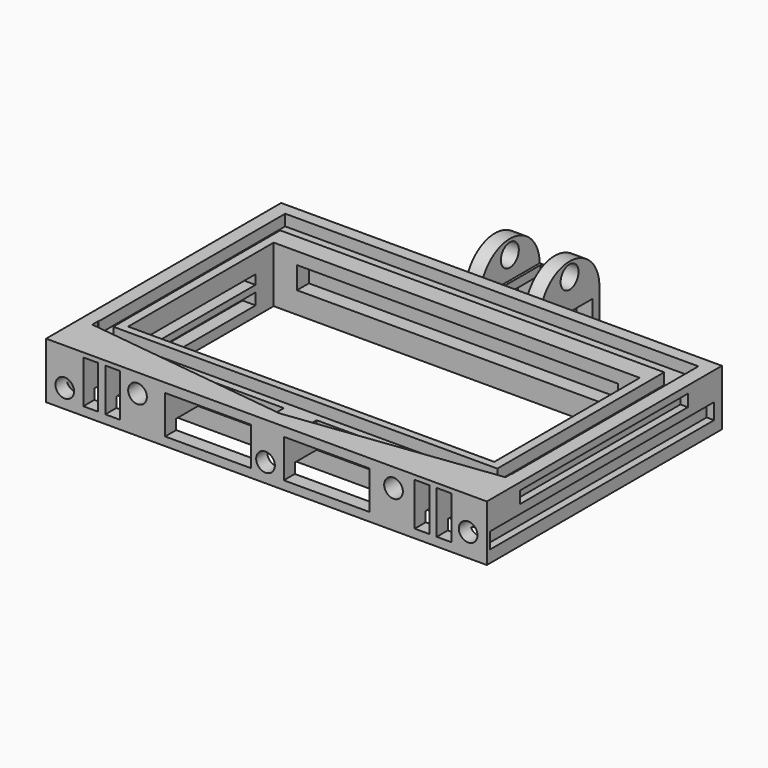
from build123d import *

# Parameters (mm, degrees)
F0_W      = 124.6
F0_H      = 61.9
F1_DEPTH  = 19.05
F2_W      = 4.953
F2_H      = 14.6315630991
F2_W_2    = 29.2449435338
F2_H_2    = 13.041177066
F2_W_3    = 29.159436468
F2_R      = 3.175
F3_DEPTH  = 13.97
F5_DEPTH  = 6.35
F6_W      = 12.7
F6_H      = 25.4
F7_DEPTH  = 12.7
F8_W      = 4.953
F8_H      = 71.0073517896
F9_DEPTH  = 3.81
F10_R     = 3.81
F11_DEPTH = 5.08
F13_DEPTH = 5.08
F14_DEPTH = 31.75
F16_W     = 13.5046280921
F16_H     = 23.5811583698
F17_DEPTH = 25.4
F18_W     = 19.2745104432
F18_H     = 5.7546193711
F19_DEPTH = 31.75
F20_W     = 14.9206416681
F20_H     = 4.7117811628
F21_DEPTH = 19.05
F22_W     = 51.0552711785
F22_H     = 10.1753515191
F22_W_2   = 51.412301138
F23_DEPTH = 12.7
F24_W     = 93.4092327952
F24_H     = 5.8380772825
F24_W_2   = 76.4692127705
F24_H_2   = 3.4473836422
F25_DEPTH = 2.54
F26_W     = 95.3170992434
F26_H     = 5.4240481682
F26_W_2   = 71.3913366199
F26_H_2   = 4.0845796466
F27_DEPTH = 2.54
F28_W     = 109.2679016292
F28_H     = 7.5388159603
F29_DEPTH = 5.08
F30_W     = 48.6481711268
F30_H     = 3.1835205168
F30_W_2   = 48.6969016492
F30_H_2   = 3.9205837529
F31_DEPTH = 5.08
F32_W     = 55.2894864231
F32_H     = 4.0775961243
F32_W_2   = 55.2933309227
F32_H_2   = 3.075633198
F33_DEPTH = 5.08


# Not quite as in the source:
# - a feature names something its author has since deleted; it is built from what else it names


with BuildPart() as f1:
    # F0 (on Top) → F1 (new body)
    with BuildSketch(Plane.XY):
        Polygon((-75.2904937168, 49.9057597088), (-75.2904937168, -50.0942402912), (-42.6597435957, -50.0942402912), (67.6151300783, -50.0942402912), (74.7095062832, -50.0942402912), (74.7095062832, 49.9057597088), (-0.2904937168, 49.9057597088), (-25.810170721, 49.9057597088), (-50.4447113996, 49.9057597088), align=None)
        with Locations((-0.2904937168, -0.0942402912)):
            Rectangle(F0_W, F0_H, mode=Mode.SUBTRACT)
    extrude(amount=F1_DEPTH)

    # F2 (on face) → F3 (cut)
    with BuildSketch(Plane.XZ.offset(50.0942402912)):
        with Locations((-60.1431414232, 10.2322226157)):
            Rectangle(F2_W, F2_H)
        with Locations((-52.6501414232, 10.2322226157)):
            Rectangle(F2_W, F2_H)
        with Locations((-20.147212787, 9.4370295992)):
            Rectangle(F2_W_2, F2_H_2)
        with Locations((20.1876896899, 9.4370295992)):
            Rectangle(F2_W_3, F2_H_2)
        with Locations((52.6363079239, 10.2322226157)):
            Rectangle(F2_W, F2_H)
        with Locations((60.1293079239, 10.2322226157)):
            Rectangle(F2_W, F2_H)
        with Locations((-44.1754937168, 12.7)):
            Circle(F2_R)
        with Locations((-0.6144937168, 6.35)):
            Circle(F2_R)
        with Locations((42.9465062832, 12.7)):
            Circle(F2_R)
        with Locations((68.3465062832, 7.8599134153)):
            Circle(F2_R)
        with Locations((-68.9404937168, 6.35)):
            Circle(F2_R)
    extrude(amount=-F3_DEPTH, mode=Mode.SUBTRACT)

    # F4 (on face) → F5 (cut)
    with BuildSketch(Plane(origin=(0, 0, 0), x_dir=(1, 0, 0), z_dir=(0, 0, -1))):
        Polygon((66.3145062832, 45.4020188174), (-67.0354937168, 45.4020188174), (-67.0354937168, 35.2429834301), (-61.1156715149, 35.2429834301), (60.9613691041, 35.2429834301), (66.3145062832, 35.2429834301), align=None)
        Polygon((-67.0354937168, 35.2429834301), (-67.0354937168, 45.4020188174), (-71.9995722175, 45.4020188174), (-71.9995722175, -45.2067597088), (-67.0354937168, -45.2067597088), (-67.0354937168, -35.52858904), align=None)
        Polygon((71.2675062832, 45.4020188174), (66.3145062832, 45.4020188174), (66.3145062832, 35.2429834301), (66.4545062832, 35.2429834301), (66.4545062832, -35.52858904), (66.4545062832, -45.2067597088), (71.2675062832, -45.2067597088), align=None)
        Polygon((60.9613691041, -35.52858904), (-67.0354937168, -35.52858904), (-67.0354937168, -45.2067597088), (66.4545062832, -45.2067597088), (66.4545062832, -35.52858904), align=None)
    extrude(amount=-F5_DEPTH, mode=Mode.SUBTRACT)

    # F6 (on face) → F7 (join)
    with BuildSketch(Plane(origin=(0, 0, 0), x_dir=(1, 0, 0), z_dir=(0, 0, -1))):
        with Locations((6.35, -62.6057597088)):
            Rectangle(F6_W, F6_H)
        with Locations((-6.35, -62.6057597088)):
            Rectangle(F6_W, F6_H)
    extrude(amount=-F7_DEPTH)

    # F8 (on face) → F9 (cut)
    with BuildSketch(Plane.XY.offset(19.05)):
        Polygon((70.0243711472, 45.754622668), (-70.5914937168, 45.754622668), (-70.5914937168, 37.4231114984), (-65.6384937168, 37.4231114984), (65.065138042, 37.4231114984), (70.0243711472, 37.4231114984), align=None)
        with Locations((-68.1149937168, 1.9194356036)):
            Rectangle(F8_W, F8_H)
        Polygon((70.0243711472, -33.5842402912), (70.0243711472, 37.4231114984), (65.065138042, 37.4231114984), (65.065138042, -33.5842402912), (69.871573916, -33.5842402912), align=None)
        Polygon((-65.6384937168, -33.5842402912), (-70.5914937168, -33.5842402912), (-70.7442909479, -33.5842402912), (-70.7442909479, -36.1242402912), (69.871573916, -36.1242402912), (69.871573916, -33.5842402912), (65.065138042, -33.5842402912), align=None)
        Polygon((69.871573916, -36.1242402912), (-70.7442909479, -36.1242402912), (0, -44.9241176248), align=None)
    extrude(amount=-F9_DEPTH, mode=Mode.SUBTRACT)

    # F10 (on face) → F11 (join)
    with BuildSketch(Plane.YZ.offset(12.7)):
        with BuildLine():
            Line((49.9057597088, 12.7), (75.3057597088, 12.7))
            ThreePointArc((75.3057597088, 12.7), (62.6057597088, 25.0247137147), (49.9057597088, 12.7))
        make_face()
        with Locations((62.6057597088, 20.32)):
            Circle(F10_R, mode=Mode.SUBTRACT)
        with Locations((62.6057597088, 20.32)):
            Circle(F10_R)
    extrude(amount=-F11_DEPTH)

    # F12 (on face) → F13 (join)
    with BuildSketch(Plane(origin=(-12.7, 0, 0), x_dir=(0, -1, 0), z_dir=(-1, 0, 0))):
        with BuildLine():
            Line((-75.3057597088, 12.7), (-49.9057597088, 12.7))
            ThreePointArc((-49.9057597088, 12.7), (-62.6057597088, 25.1906117041), (-75.3057597088, 12.7))
        make_face()
    extrude(amount=-F13_DEPTH)

    # F10 (on face) → F14 (cut)
    with BuildSketch(Plane.YZ.offset(12.7)):
        with Locations((62.6057597088, 20.32)):
            Circle(F10_R)
    extrude(amount=-F14_DEPTH, mode=Mode.SUBTRACT)

    # F16 (on face) → F17 (cut)
    with BuildSketch(Plane.XY.offset(12.7)):
        with Locations((-0.017571263, 62.7732072026)):
            Rectangle(F16_W, F16_H)
    extrude(amount=-F17_DEPTH, mode=Mode.SUBTRACT)

    # F18 (on face) → F19 (cut)
    with BuildSketch(Plane(origin=(-12.7, 0, 0), x_dir=(0, -1, 0), z_dir=(-1, 0, 0))):
        with Locations((-62.7002157271, 6.9401275832)):
            Rectangle(F18_W, F18_H)
    extrude(amount=-F19_DEPTH, mode=Mode.SUBTRACT)

    # F20 (on face) → F21 (cut)
    with BuildSketch(Plane(origin=(0, 75.3057597088, 0), x_dir=(-1, 0, 0), z_dir=(0, 1, 0))):
        with Locations((0.1047314145, 6.2031324487)):
            Rectangle(F20_W, F20_H)
    extrude(amount=-F21_DEPTH, mode=Mode.SUBTRACT)

    # F22 (on face) → F23 (cut)
    with BuildSketch(Plane(origin=(0, 49.9057597088, 0), x_dir=(-1, 0, 0), z_dir=(0, 1, 0))):
        with Locations((-43.9973082393, 9.4878289383)):
            Rectangle(F22_W, F22_H)
        with Locations((44.010556303, 9.4878289383)):
            Rectangle(F22_W_2, F22_H)
    extrude(amount=-F23_DEPTH, mode=Mode.SUBTRACT)

    # F24 (on face) → F25 (cut)
    with BuildSketch(Plane(origin=(-75.2904937168, 0, 0), x_dir=(0, -1, 0), z_dir=(-1, 0, 0))):
        with Locations((0.03618747, 6.7635682644)):
            Rectangle(F24_W, F24_H)
        with Locations((0.2549141645, 13.9791369438)):
            Rectangle(F24_W_2, F24_H_2)
    extrude(amount=-F25_DEPTH, mode=Mode.SUBTRACT)

    # F26 (on face) → F27 (cut)
    with BuildSketch(Plane.YZ.offset(74.7095062832)):
        with Locations((-1.0910946876, 6.8129759159)):
            Rectangle(F26_W, F26_H)
        with Locations((-0.289645046, 14.5612489432)):
            Rectangle(F26_W_2, F26_H_2)
    extrude(amount=-F27_DEPTH, mode=Mode.SUBTRACT)

    # F28 (on face) → F29 (cut)
    with BuildSketch(Plane.XZ.offset(-30.8557597088)):
        with Locations((-0.0406969339, 11.1216651276)):
            Rectangle(F28_W, F28_H)
    extrude(amount=-F29_DEPTH, mode=Mode.SUBTRACT)

    # F30 (on face) → F31 (cut)
    with BuildSketch(Plane.YZ.offset(-62.5904937168)):
        with Locations((-1.1887364089, 11.1167602584)):
            Rectangle(F30_W, F30_H)
        with Locations((-1.1643711478, 5.3142114775)):
            Rectangle(F30_W_2, F30_H_2)
    extrude(amount=-F31_DEPTH, mode=Mode.SUBTRACT)

    # F32 (on face) → F33 (cut)
    with BuildSketch(Plane(origin=(62.0095062832, 0, 0), x_dir=(0, -1, 0), z_dir=(-1, 0, 0))):
        with Locations((1.1272905394, 6.7439966369)):
            Rectangle(F32_W, F32_H)
        with Locations((1.1480180547, 12.1434889734)):
            Rectangle(F32_W_2, F32_H_2)
    extrude(amount=-F33_DEPTH, mode=Mode.SUBTRACT)


solid = f1.part
